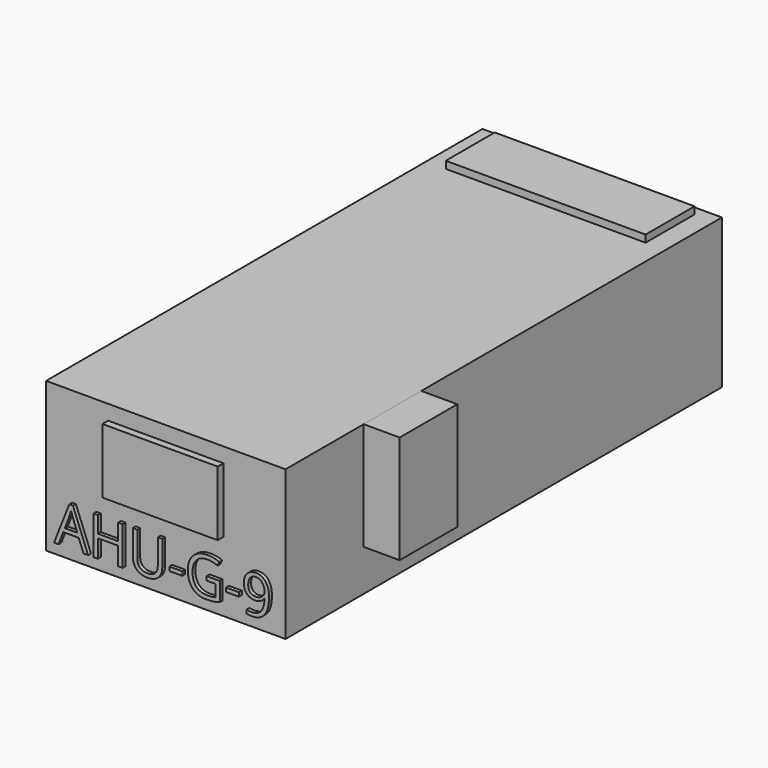
from build123d import *

# Parameters (mm, degrees)
F0_W         = 1689.1
F0_H         = 1054.1
F1_DEPTH     = 3848.1
F2_W         = 812.8
F2_H         = 457.2
F3_DEPTH     = 50.8
F4_W         = 508
F4_H         = 762
F5_DEPTH     = 254
F6_TEXT_SIZE = 380.2978537149
F7_DEPTH     = 25.4
F8_W         = 1409.7
F8_H         = 431.8
F9_DEPTH     = 50.8
F10_W        = 1409.7
F10_H        = 431.8
F11_DEPTH    = 50.8


# Not quite as in the source:
# - Text() gives the source's letters only with a copy of the font that has no kerning and outlines rounded to 1/6400 em; it was checked with that copy


with BuildPart() as f1:
    # F0 (on Front) → F1 (new body)
    with BuildSketch(Plane.XZ):
        with Locations((204.6098696411, -25.3882179465)):
            Rectangle(F0_W, F0_H)
    extrude(amount=F1_DEPTH)

    # F2 (on face) → F3 (join)
    with BuildSketch(Plane.XZ.offset(3848.1)):
        with Locations((204.6098696411, 168.2867820535)):
            Rectangle(F2_W, F2_H)
    extrude(amount=F3_DEPTH)

    # F6 (on face) → F7 (join)
    with BuildSketch(Plane.XZ.offset(3848.1)):
        with Locations((-563.5762512684, -467.682570219)):
            Text('AHU-G-9', F6_TEXT_SIZE, font='Open Sans', text_align=(TextAlign.LEFT, TextAlign.BOTTOM))
    extrude(amount=F7_DEPTH)

    # F8 (on face) → F9 (join)
    with BuildSketch(Plane(origin=(0, 0, 0), x_dir=(-1, 0, 0), z_dir=(0, 1, 0))):
        with Locations((-204.6098696411, 9.5367820535)):
            Rectangle(F8_W, F8_H)
    extrude(amount=F9_DEPTH)

    # F10 (on face) → F11 (join)
    with BuildSketch(Plane.XY.offset(501.6617820535)):
        with Locations((204.6098696411, -282.575)):
            Rectangle(F10_W, F10_H)
    extrude(amount=F11_DEPTH)


with BuildPart() as f5:
    # F4 (on face) → F5 (new body)
    with BuildSketch(Plane.YZ.offset(1049.1598696411)):
        with Locations((-2905.125, 120.6617820535)):
            Rectangle(F4_W, F4_H)
    extrude(amount=F5_DEPTH)


solid = Compound([f1.part, f5.part])
